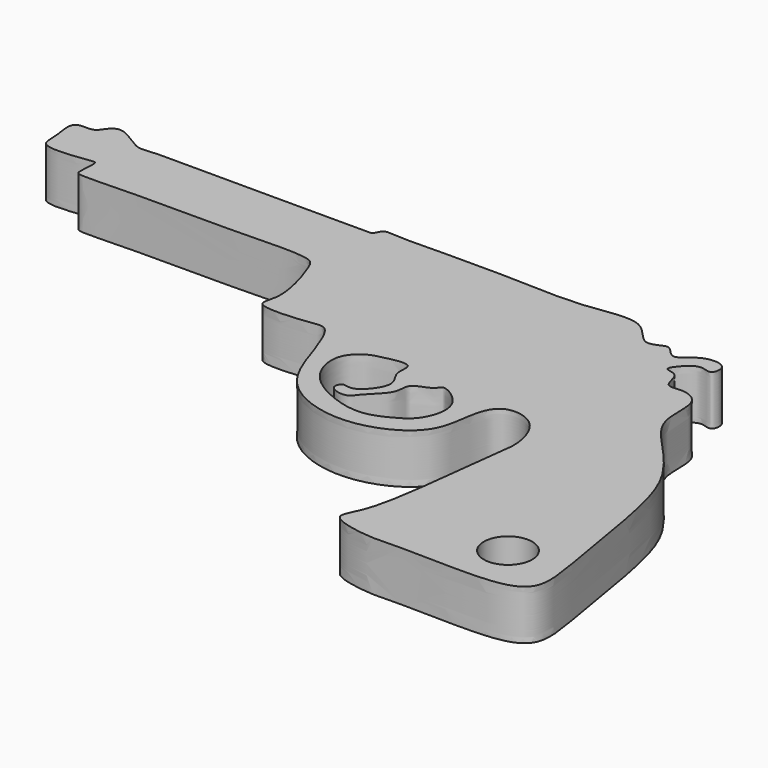
from build123d import *

# Parameters (mm, degrees)
F0_R     = 2.9147006616
F1_DEPTH = 6


# Not quite as in the source:
# - the program builds the solid bodies; features that only make, move or delete a surface that nothing else refers to are left out


with BuildPart() as f1:
    # F0 (on Top) → F1 (new body)
    with BuildSketch(Plane.XY):
        with BuildLine():
            add(Edge.make_bspline(
                [(-49.6023209556, 18.0272394648), (-49.8074049045, 18.1029147074), (-50.0135140203, 18.4552867998), (-49.6134118775, 20.9119208188), (-50.5253484682, 20.8059587598), (-56.4945372814, 19.9108445595), (-55.9537471934, 22.5685842047), (-56.9971661783, 26.2589865372), (-54.0763480855, 25.5348560374), (-53.4557302149, 26.7840339255), (-52.0635197146, 28.1049552213), (-48.8894052923, 25.4511846491), (-47.3733605364, 25.8661869079), (-40.4968760467, 25.7376088359), (-29.8507681218, 25.8091465961), (-21.0487484491, 25.7490835391), (-20.4024617931, 25.8118263554), (-20.0328825434, 27.0620609399), (-18.1976358309, 26.6124423912), (-6.9570984973, 27.1733866362), (3.8117240872, 26.2249589242), (10.9843657407, 28.2020637076), (13.1552615006, 23.7187810056), (15.3714876777, 25.2903636303), (16.136817469, 24.9800189126), (17.4081822679, 23.1858848474), (19.2613078068, 25.8045591801), (22.6884322766, 25.6811552369), (22.2588685569, 23.0964670957), (20.558135038, 24.2612231235), (18.9074395708, 22.7290362197), (18.0319969708, 21.3185632856), (20.1574134565, 21.4939458775), (20.1690381309, 18.5500576059), (22.2769119615, 19.2643947473), (25.1306908499, 18.1604015194), (24.2741164567, 13.2326866853), (27.0607669188, 9.7406518128), (32.4347089231, 4.3395026277), (34.4573175975, -3.9334445072), (36.1279143933, -14.5901637251), (37.3183979381, -21.4880036609), (31.6796050531, -22.9715878156), (22.3026977732, -22.3468961354), (18.0434343424, -22.8509233977), (12.0162311177, -21.6154183479), (14.901467169, -18.365273499), (15.9808130291, -6.0483306163), (16.666526274, -1.8712639675), (17.1011194141, 1.4668769818), (15.4325203205, 5.6829770649), (10.8625859398, 6.2372133359), (9.6626017816, 2.3361906801), (9.4808715441, -2.7713821565), (1.5213780842, -6.7779297446), (-7.6731415433, -3.7547507099), (-9.761336118, 3.5621435123), (-11.6495824525, 8.4220182056), (-13.7775909876, 7.8879501127), (-20.7391399513, 7.3101422928), (-18.7124742611, 10.3369667678), (-20.7645413341, 16.6669335216), (-21.8112583257, 18.4584177885), (-31.0078706979, 17.9255039273), (-44.3635723867, 18.1777572258), (-49.0263092465, 17.8146932072), (-49.6023209556, 18.0272394648)],
                knots=[0, 0, 0, 0, 0.005935078, 0.0175951552, 0.0239432968, 0.0420063258, 0.0532269701, 0.0669117352, 0.0779273846, 0.0868186658, 0.0964708455, 0.1114418033, 0.1211284516, 0.1410206824, 0.1687737919, 0.1913673607, 0.1967204234, 0.2044388586, 0.2138092055, 0.2401669057, 0.267646687, 0.2877343994, 0.3027287684, 0.3137676843, 0.320641509, 0.3304829452, 0.3433106776, 0.3562721449, 0.365809702, 0.3751082564, 0.3868053621, 0.3951079593, 0.4042295641, 0.415793231, 0.4260149386, 0.4384195025, 0.454817304, 0.4713696863, 0.4928203417, 0.5161102815, 0.5427723779, 0.561872532, 0.5790177112, 0.6034149628, 0.6211241043, 0.637886273, 0.6513113797, 0.6794406659, 0.6962994492, 0.7103888721, 0.726529859, 0.7413322318, 0.7559839172, 0.7732983638, 0.7954867055, 0.8188633052, 0.8405839663, 0.8572615179, 0.868582535, 0.8873461566, 0.8989460787, 0.9192697971, 0.9297097593, 0.9527613841, 0.9833303657, 1, 1, 1, 1], degree=3))
        make_face()
        with Locations((29.8542086492, -16.7032843149)):
            Circle(F0_R, mode=Mode.SUBTRACT)
        with BuildLine():
            add(Edge.make_bspline(
                [(-1.0609307354, 6.8363510625), (-1.4873269942, 7.249000096), (-4.0736565125, 6.6621158658), (-5.745052855, 6.2437274615), (-7.8877921378, 4.0934006501), (-6.6874148039, -0.5681944173), (-1.8998880071, -3.0434868049), (1.7595930368, -3.6404349466), (4.6556018883, -2.2523534565), (6.8122191281, -0.9145123394), (8.161197299, 3.4853110891), (4.1281422183, 6.0229396454), (3.9586665615, 4.5636478818), (1.1522679825, 4.0853638837), (1.7753034047, 1.7483239013), (-0.9525375044, -0.3797461415), (-1.5515597494, -1.8192513773), (-4.1832932305, -1.2926465042), (-3.5226896431, 0.4136772132), (-2.0243664942, -0.6508577164), (0.9505711019, 2.9997561949), (-1.3383084002, 4.7818012859), (-0.7181969406, 6.5046671739), (-1.0609307354, 6.8363510625)],
                knots=[0, 0, 0, 0, 0.0504856732, 0.0929388967, 0.1408080364, 0.2024445263, 0.2714031111, 0.3288549318, 0.3810507153, 0.4288190471, 0.4888951383, 0.5450438002, 0.5728202259, 0.6182182572, 0.659337254, 0.7134296933, 0.749891138, 0.7919053815, 0.8220077903, 0.8559448629, 0.9130707698, 0.9594200324, 1, 1, 1, 1], degree=3))
        make_face(mode=Mode.SUBTRACT)
    extrude(amount=F1_DEPTH)


solid = f1.part
